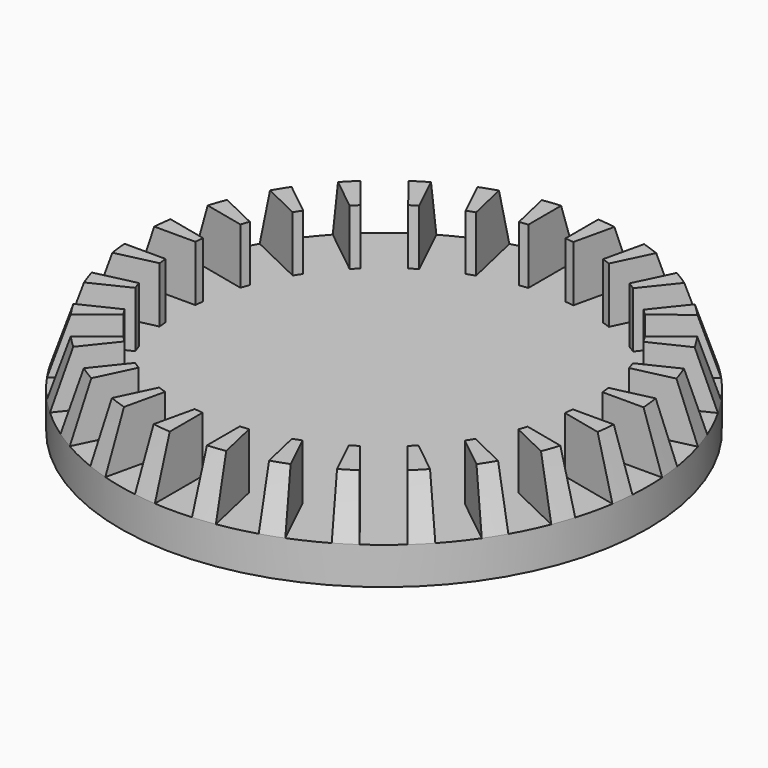
from build123d import *

# Parameters (mm, degrees)
F0_R            = 71
F1_DEPTH        = 25
F2_SIZE2        = 15
F2_SIZE         = 5
F3_R            = 55
F4_DEPTH        = 15
F5_W            = 10
F5_H            = 20
F6_DEPTH        = 114.4
F6_COPIES_COUNT = 28


# Not quite as in the source:
# - a pattern or mirror of a feature is missing from the dataset's text; its kind, count and spacing are read off the source's solid


with BuildPart() as f1:
    # F0 (on Top) → F1 (new body)
    with BuildSketch(Plane.XY):
        Circle(F0_R)
    extrude(amount=F1_DEPTH)

    # F2
    f2_edges = [f1.edges().sort_by_distance(p)[0] for p in [
        (-71, 0, 25),
    ]]
    f2_side = f1.faces().sort_by_distance((0, 0, 25))[0]
    chamfer(f2_edges, length=F2_SIZE, length2=F2_SIZE2, reference=f2_side)

    # F3 (on face) → F4 (cut)
    with BuildSketch(Plane.XY.offset(25)):
        Circle(F3_R)
    extrude(amount=-F4_DEPTH, mode=Mode.SUBTRACT)

    # F5 (on Front) → F6 (cut)
    with BuildSketch(Plane.XZ):
        with Locations((0, 20)):
            Rectangle(F5_W, F5_H)
    f6 = extrude(amount=F6_DEPTH, mode=Mode.SUBTRACT)

    # F6_copies: F6 ×28 about axis
    f6_copies_axis = Axis((0, 0, 0), (0, 0, 1))
    for i in range(1, F6_COPIES_COUNT):
        add(f6.rotate(f6_copies_axis, i * 360 / F6_COPIES_COUNT), mode=Mode.SUBTRACT)


solid = f1.part
